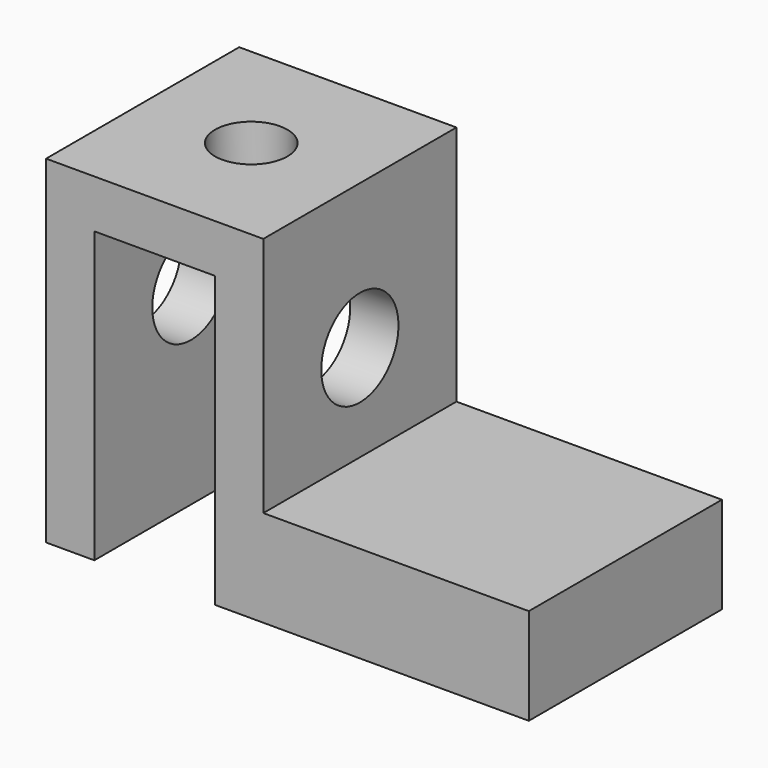
from build123d import *

# Parameters (mm, degrees)
F0_W      = 100
F0_H      = 50
F1_DEPTH  = 20
F2_W      = 45
F2_H      = 50
F3_DEPTH  = 50
F4_W      = 25
F4_H      = 60
F5_DEPTH  = 50.001
F6_R      = 10
F7_DEPTH  = 100.001
F8_R      = 7.5
F10_DEPTH = 70.001


# Not quite as in the source:
# - a feature of the source that left no trace in its solid (it failed there, or was rolled back) is left out


with BuildPart() as f1:
    # F0 (on Top) → F1 (new body)
    with BuildSketch(Plane.XY):
        with Locations((50, 25)):
            Rectangle(F0_W, F0_H)
    extrude(amount=F1_DEPTH)

    # F2 (on face) → F3 (join)
    with BuildSketch(Plane.XY.offset(20)):
        with Locations((22.5, 25)):
            Rectangle(F2_W, F2_H)
    extrude(amount=F3_DEPTH)

    # F4 (on face) → F5 (cut, through all)
    with BuildSketch(Plane.XZ):
        with Locations((22.5, 30)):
            Rectangle(F4_W, F4_H)
    extrude(amount=-F5_DEPTH, mode=Mode.SUBTRACT)

    # F6 (on face) → F7 (cut, through all)
    with BuildSketch(Plane(origin=(0, 0, 0), x_dir=(0, -1, 0), z_dir=(-1, 0, 0))):
        with Locations((-25, 40)):
            Circle(F6_R)
    extrude(amount=-F7_DEPTH, mode=Mode.SUBTRACT)

    # F8 (on face) → F10 (cut, through all)
    with BuildSketch(Plane.XY.offset(70)):
        with Locations((22.5, 25)):
            Circle(F8_R)
    extrude(amount=-F10_DEPTH, mode=Mode.SUBTRACT)


solid = f1.part
